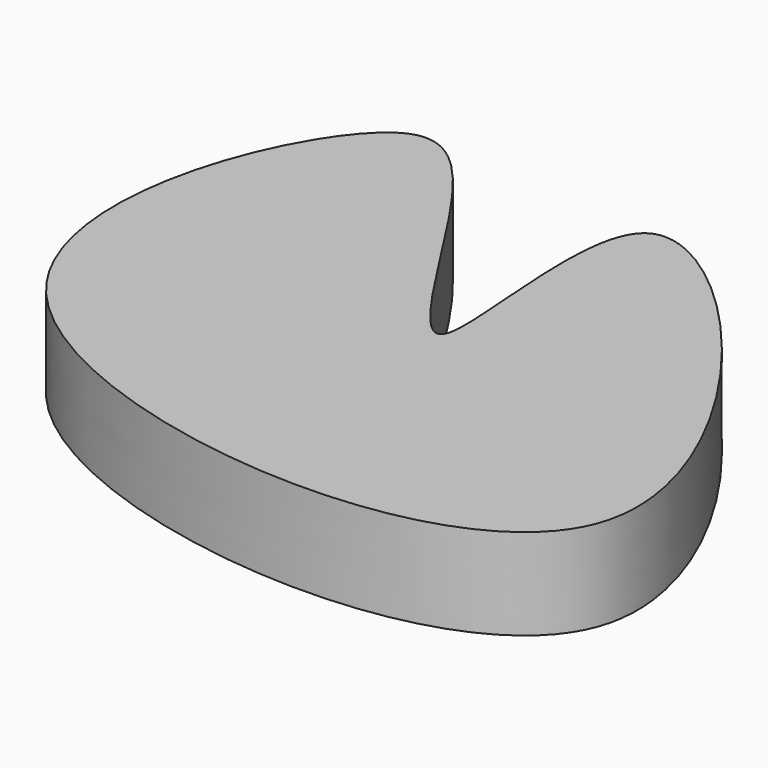
from build123d import *

# Parameters (mm, degrees)
F1_DEPTH = 25.4


# Not quite as in the source:
# - the program builds the solid bodies; features that only make, move or delete a surface that nothing else refers to are left out


with BuildPart() as f1:
    # F0 (on Top) → F1 (new body)
    with BuildSketch(Plane.XY):
        with BuildLine():
            add(Edge.make_bspline(
                [(-89.3034636974, 77.5415599346), (-106.1213513806, 62.1554739644), (-153.5112654022, -61.5579093212), (153.2228761671, -87.0037013585), (-43.8815566445, 145.3380521797), (-1.7070066843, -37.4716393849), (-61.1809052267, 79.1574417961), (-80.8703775867, 85.2566898212), (-89.3034636974, 77.5415599346)],
                knots=[0, 0, 0, 0, 0.1812334503, 0.406708922, 0.6134849908, 0.7566224491, 0.9091231122, 1, 1, 1, 1], degree=3))
        make_face()
    extrude(amount=F1_DEPTH)


solid = f1.part
